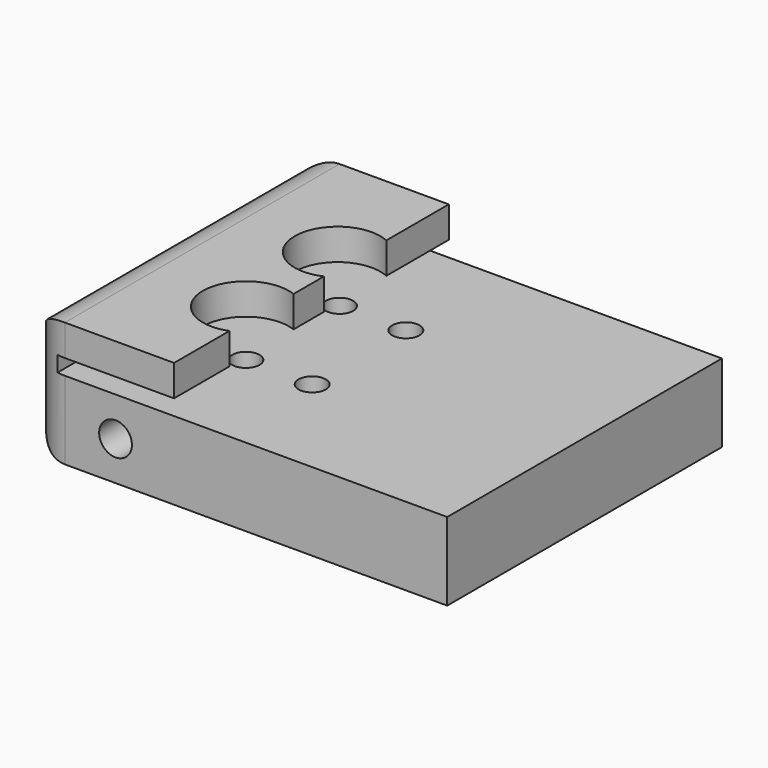
from build123d import *

# Parameters (mm, degrees)
F0_W         = 15
F0_H         = 4
F1_DEPTH     = 44
F3_D         = 3.5
F4_R         = 1.75
F5_DEPTH     = 4
F7_D         = 4.2
F9_D         = 3.5
F9_DEPTH     = 10.001
F11_DEPTH    = 4
F12_T1_DEPTH = 69
F12_T3_DEPTH = 41


# Not quite as in the source:
# - a fillet or chamfer that OpenCascade refuses, or shapes differently, is made with other operations: its cross-section is extruded or revolved along the edge and cut away or added


with BuildPart() as f1:
    # F0 (on Front) → F1 (new body)
    with BuildSketch(Plane.XZ):
        Polygon((-28.8571389138, 6), (-28.8571389138, 0), (-24.8571389138, 0), (-24.8571389138, 2), (-24.8571389138, 6), align=None)
        Polygon((-24.8571389138, 0), (-28.8571389138, 0), (-28.8571389138, -10), (25.1428610862, -10), (25.1428610862, 0), align=None)
        with Locations((-17.3571389138, 4)):
            Rectangle(F0_W, F0_H)
    extrude(amount=F1_DEPTH)

    # F3 (through all)
    with Locations(Plane(origin=(0, 0, -10), x_dir=(1, 0, 0), z_dir=(0, 0, -1))):
        with Locations((-11.8571389138, 15), (-3.3571389138, 30)):
            Hole(F3_D / 2)

    # F4 (on face) → F5 (cut)
    with BuildSketch(Plane.XY.offset(6)):
        with BuildLine():
            Line((-9.8571389138, -20), (-9.8571389138, -10))
            ThreePointArc((-9.8571389138, -10), (-17.5900669637, -15), (-9.8571389138, -20))
        make_face()
        with Locations((-11.8571389138, -15)):
            Circle(F4_R, mode=Mode.SUBTRACT)
    extrude(amount=-F5_DEPTH, mode=Mode.SUBTRACT)

    # F7 (through all)
    with Locations(Plane.XZ.offset(44)):
        with Locations((-17.3571389138, -5)):
            Hole(F7_D / 2)

    # F9 (through all, one way)
    with BuildSketch(Plane.XY):
        with Locations((-3.3571389138, -15), (-11.8571389138, -30)):
            Circle(F9_D / 2)
    extrude(amount=-F9_DEPTH, mode=Mode.SUBTRACT)

    # F10 (on face) → F11 (cut, through all)
    with BuildSketch(Plane.XY.offset(6)):
        with BuildLine():
            Line((-9.8571389138, -35.1305356622), (-9.8571389138, -24.8694643378))
            ThreePointArc((-9.8571389138, -24.8694643378), (-17.3637164517, -30), (-9.8571389138, -35.1305356622))
        make_face()
    extrude(amount=-F11_DEPTH, mode=Mode.SUBTRACT)

    # F12: fillet of radius 5 on 4 edges, made by hand

    # F12_s2 → F12_t1 (cut)
    with BuildSketch(Plane.XZ.offset(-12.5)):
        with BuildLine():
            ThreePointArc((-28.8571389138, 1), (-27.3926728198, 4.5355339059), (-23.8571389138, 6))
            Line((-23.8571389138, 6), (-28.8571389138, 6))
            Line((-28.8571389138, 6), (-28.8571389138, 1))
        make_face()
        with BuildLine():
            ThreePointArc((-28.8571389138, -5), (-27.3926728198, -8.5355339059), (-23.8571389138, -10))
            Line((-23.8571389138, -10), (-28.8571389138, -10))
            Line((-28.8571389138, -10), (-28.8571389138, -5))
        make_face()
    extrude(amount=F12_T1_DEPTH, mode=Mode.SUBTRACT)

    # F12_s4 → F12_t3 (cut)
    with BuildSketch(Plane.XY.offset(-22.5)):
        with BuildLine():
            ThreePointArc((-28.8571389138, -5), (-27.3926728198, -1.4644660941), (-23.8571389138, 0))
            Line((-23.8571389138, 0), (-28.8571389138, 0))
            Line((-28.8571389138, 0), (-28.8571389138, -5))
        make_face()
        with BuildLine():
            ThreePointArc((-28.8571389138, -39), (-27.3926728198, -42.5355339059), (-23.8571389138, -44))
            Line((-23.8571389138, -44), (-28.8571389138, -44))
            Line((-28.8571389138, -44), (-28.8571389138, -39))
        make_face()
    extrude(amount=F12_T3_DEPTH, mode=Mode.SUBTRACT)


solid = f1.part
